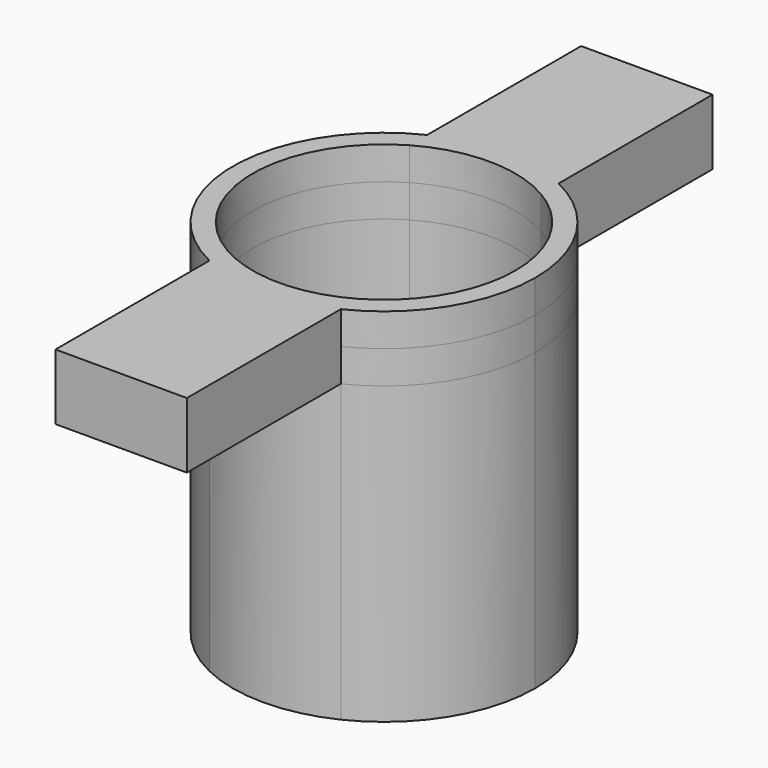
from build123d import *

# Parameters (mm, degrees)
F1_DEPTH = 10
F2_DEPTH = 1


# Not quite as in the source:
# - a feature names something its author has since deleted; it is built from what else it names


with BuildPart() as f1:
    # F0 (on Top) → F1 (new body)
    with BuildSketch(Plane.XY):
        with BuildLine():
            Line((-2, 3.4641016151), (-2, 4.1424630354))
            ThreePointArc((-2, 4.1424630354), (-4.6, 0), (-2, -4.1424630354))
            Line((-2, -4.1424630354), (-2, -3.4641016151))
            ThreePointArc((-2, -3.4641016151), (-4, 0), (-2, 3.4641016151))
        make_face()
        with BuildLine():
            ThreePointArc((-2, -4.1424630354), (0, -4.6), (2, -4.1424630354))
            Line((2, -4.1424630354), (2, -3.4641016151))
            ThreePointArc((2, -3.4641016151), (0, -4), (-2, -3.4641016151))
            Line((-2, -3.4641016151), (-2, -4.1424630354))
        make_face()
        with BuildLine():
            ThreePointArc((2, -4.1424630354), (3.8961519478, -2.4454038521), (4.6, 0))
            ThreePointArc((4.6, 0), (3.8961519478, 2.4454038521), (2, 4.1424630354))
            Line((2, 4.1424630354), (2, 3.4641016151))
            ThreePointArc((2, 3.4641016151), (3.4641016151, 2), (4, 0))
            ThreePointArc((4, 0), (3.4641016151, -2), (2, -3.4641016151))
            Line((2, -3.4641016151), (2, -4.1424630354))
        make_face()
        with BuildLine():
            Line((2, 3.4641016151), (2, 4.1424630354))
            ThreePointArc((2, 4.1424630354), (0, 4.6), (-2, 4.1424630354))
            Line((-2, 4.1424630354), (-2, 3.4641016151))
            ThreePointArc((-2, 3.4641016151), (0, 4), (2, 3.4641016151))
        make_face()
    extrude(amount=-F1_DEPTH)

    # F0 (on Top) → F2 (join, symmetric)
    with BuildSketch(Plane.XY):
        with BuildLine():
            ThreePointArc((-2, 4.1424630354), (0, 4.6), (2, 4.1424630354))
            Line((2, 4.1424630354), (2, 10))
            Line((2, 10), (-2, 10))
            Line((-2, 10), (-2, 4.1424630354))
        make_face()
        with BuildLine():
            Line((2, -10), (2, -4.1424630354))
            ThreePointArc((2, -4.1424630354), (0, -4.6), (-2, -4.1424630354))
            Line((-2, -4.1424630354), (-2, -10))
            Line((-2, -10), (2, -10))
        make_face()
        with BuildLine():
            Line((2, 3.4641016151), (2, 4.1424630354))
            ThreePointArc((2, 4.1424630354), (0, 4.6), (-2, 4.1424630354))
            Line((-2, 4.1424630354), (-2, 3.4641016151))
            ThreePointArc((-2, 3.4641016151), (0, 4), (2, 3.4641016151))
        make_face()
        with BuildLine():
            ThreePointArc((-2, -4.1424630354), (0, -4.6), (2, -4.1424630354))
            Line((2, -4.1424630354), (2, -3.4641016151))
            ThreePointArc((2, -3.4641016151), (0, -4), (-2, -3.4641016151))
            Line((-2, -3.4641016151), (-2, -4.1424630354))
        make_face()
        with BuildLine():
            Line((-2, 3.4641016151), (-2, 4.1424630354))
            ThreePointArc((-2, 4.1424630354), (-4.6, 0), (-2, -4.1424630354))
            Line((-2, -4.1424630354), (-2, -3.4641016151))
            ThreePointArc((-2, -3.4641016151), (-4, 0), (-2, 3.4641016151))
        make_face()
        with BuildLine():
            ThreePointArc((2, -4.1424630354), (3.8961519478, -2.4454038521), (4.6, 0))
            ThreePointArc((4.6, 0), (3.8961519478, 2.4454038521), (2, 4.1424630354))
            Line((2, 4.1424630354), (2, 3.4641016151))
            ThreePointArc((2, 3.4641016151), (3.4641016151, 2), (4, 0))
            ThreePointArc((4, 0), (3.4641016151, -2), (2, -3.4641016151))
            Line((2, -3.4641016151), (2, -4.1424630354))
        make_face()
    extrude(amount=F2_DEPTH, both=True)


solid = f1.part
